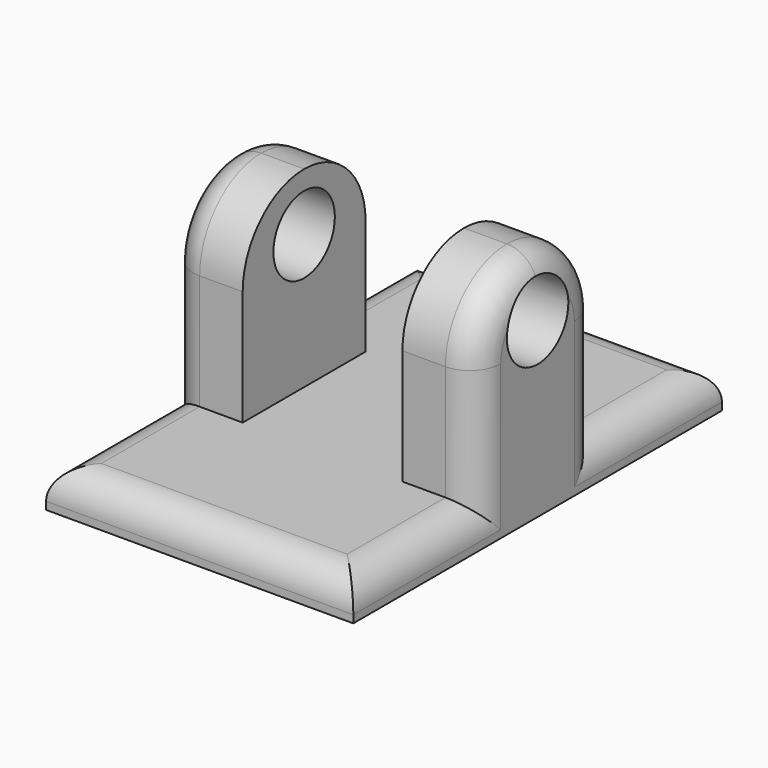
from build123d import *

# Parameters (mm, degrees)
F0_W         = 50.8
F0_H         = 76.2
F1_DEPTH     = 6.35
F2_W         = 12.192
F2_H         = 25.4
F3_DEPTH     = 31.75
F5_D         = 12.7
F5_DEPTH     = 254
F5_TIP       = 3.8154649308
F6_R         = 12.69999
F7_T1_DEPTH  = 19.05001
F7_T3_DEPTH  = 76.2
F7_T5_DEPTH  = 38.1
F7_T7_DEPTH  = 38.1
F7_T9_DEPTH  = 2e-05
F7_T12_ANGLE = 90
F7_T14_ANGLE = 90
F7_T16_ANGLE = 90
F7_T18_ANGLE = 90
F7_T23_DEPTH = 31.75001
F7_T28_DEPTH = 38.1
F7_T35_DEPTH = 38.1
F7_T39_DEPTH = 31.75001
F7_T47_DEPTH = 38.1
F7_T51_DEPTH = 31.75001
F7_T59_DEPTH = 31.75001
F7_T64_DEPTH = 38.1


# Not quite as in the source:
# - a fillet or chamfer that OpenCascade refuses, or shapes differently, is made with other operations: its cross-section is extruded or revolved along the edge and cut away or added
# - a fillet or chamfer is up to 0.001 mm smaller than in the source, because OpenCascade refuses the exact size


with BuildPart() as f1:
    # F0 (on Top) → F1 (new body)
    with BuildSketch(Plane.XY):
        Rectangle(F0_W, F0_H)
    extrude(amount=F1_DEPTH)

    # F2 (on face) → F3 (join)
    with BuildSketch(Plane.XY.offset(6.35)):
        with Locations((-19.304, 0)):
            Rectangle(F2_W, F2_H)
        with Locations((19.304, 0)):
            Rectangle(F2_W, F2_H)
    extrude(amount=F3_DEPTH)

    # F5
    with Locations(Plane(origin=(-25.4, 0, 0), x_dir=(0, -1, 0), z_dir=(-1, 0, 0))):
        with Locations((0, 28.575)):
            Hole(F5_D / 2, depth=F5_DEPTH)
            with Locations((0, 0, -(F5_DEPTH + F5_TIP / 2))):  # 118° drill point
                Cone(0, F5_D / 2, F5_TIP, mode=Mode.SUBTRACT)

    # F6 (radius 12.7 in the source; OpenCascade refuses exactly that, so slightly less here)
    f6_edges = [f1.edges().sort_by_distance(p)[0] for p in [
        (19.304, 12.7, 38.1),
        (19.304, -12.7, 38.1),
        (-19.304, 12.7, 38.1),
        (-19.304, -12.7, 38.1),
    ]]
    fillet(f6_edges, radius=F6_R)

    # F7: fillet of radius 5.08 on 14 edges, made by hand

    # F7_s2 → F7_t1 (cut)
    with BuildSketch(Plane.XY.offset(6.35)):
        with BuildLine():
            ThreePointArc((-25.4, 7.62), (-23.9121024484, 11.2121024484), (-20.32, 12.7))
            Line((-20.32, 12.7), (-25.4, 12.7))
            Line((-25.4, 12.7), (-25.4, 7.62))
        make_face()
        with BuildLine():
            ThreePointArc((25.4, -7.62), (23.9121024484, -11.2121024484), (20.32, -12.7))
            Line((20.32, -12.7), (25.4, -12.7))
            Line((25.4, -12.7), (25.4, -7.62))
        make_face()
        with BuildLine():
            ThreePointArc((-25.4, -7.62), (-23.9121024484, -11.2121024484), (-20.32, -12.7))
            Line((-20.32, -12.7), (-25.4, -12.7))
            Line((-25.4, -12.7), (-25.4, -7.62))
        make_face()
        with BuildLine():
            ThreePointArc((25.4, 7.62), (23.9121024484, 11.2121024484), (20.32, 12.7))
            Line((20.32, 12.7), (25.4, 12.7))
            Line((25.4, 12.7), (25.4, 7.62))
        make_face()
    extrude(amount=F7_T1_DEPTH, mode=Mode.SUBTRACT)

    # F7_s4 → F7_t3 (cut)
    with BuildSketch(Plane.YZ.offset(-38.1)):
        with BuildLine():
            ThreePointArc((-33.02, 6.35), (-36.6121024484, 4.8621024484), (-38.1, 1.27))
            Line((-38.1, 1.27), (-38.1, 6.35))
            Line((-38.1, 6.35), (-33.02, 6.35))
        make_face()
        with BuildLine():
            ThreePointArc((33.02, 6.35), (36.6121024484, 4.8621024484), (38.1, 1.27))
            Line((38.1, 1.27), (38.1, 6.35))
            Line((38.1, 6.35), (33.02, 6.35))
        make_face()
    extrude(amount=F7_T3_DEPTH, mode=Mode.SUBTRACT)

    # F7_s6 → F7_t5 (cut)
    with BuildSketch(Plane.XZ.offset(12.7)):
        with BuildLine():
            ThreePointArc((20.32, 6.35), (23.9121024484, 4.8621024484), (25.4, 1.27))
            Line((25.4, 1.27), (25.4, 6.35))
            Line((25.4, 6.35), (20.32, 6.35))
        make_face()
        with BuildLine():
            ThreePointArc((-25.4, 1.27), (-23.9121024484, 4.8621024484), (-20.32, 6.35))
            Line((-20.32, 6.35), (-25.4, 6.35))
            Line((-25.4, 6.35), (-25.4, 1.27))
        make_face()
    extrude(amount=F7_T5_DEPTH, mode=Mode.SUBTRACT)

    # F7_s8 → F7_t7 (cut)
    with BuildSketch(Plane.XZ.offset(-50.8)):
        with BuildLine():
            ThreePointArc((20.32, 6.35), (23.9121024484, 4.8621024484), (25.4, 1.27))
            Line((25.4, 1.27), (25.4, 6.35))
            Line((25.4, 6.35), (20.32, 6.35))
        make_face()
        with BuildLine():
            ThreePointArc((-25.4, 1.27), (-23.9121024484, 4.8621024484), (-20.32, 6.35))
            Line((-20.32, 6.35), (-25.4, 6.35))
            Line((-25.4, 6.35), (-25.4, 1.27))
        make_face()
    extrude(amount=F7_T7_DEPTH, mode=Mode.SUBTRACT)

    # F7_s10 → F7_t9 (cut)
    with BuildSketch(Plane.XZ.offset(-1e-05)):
        with BuildLine():
            ThreePointArc((25.4, 33.02), (23.9121024484, 36.6121024484), (20.32, 38.1))
            Line((20.32, 38.1), (25.4, 38.1))
            Line((25.4, 38.1), (25.4, 33.02))
        make_face()
        with BuildLine():
            ThreePointArc((-25.4, 33.02), (-23.9121024484, 36.6121024484), (-20.32, 38.1))
            Line((-20.32, 38.1), (-25.4, 38.1))
            Line((-25.4, 38.1), (-25.4, 33.02))
        make_face()
    extrude(amount=F7_T9_DEPTH, mode=Mode.SUBTRACT)

    # F7_s11 → F7_t12 (revolve, cut)
    with BuildSketch(Plane.XY.offset(25.40001)):
        with BuildLine():
            ThreePointArc((-25.4, 7.62), (-23.9121024484, 11.2121024484), (-20.32, 12.7))
            Line((-20.32, 12.7), (-25.4, 12.7))
            Line((-25.4, 12.7), (-25.4, 7.62))
        make_face()
    revolve(axis=Axis((-25.4, 1e-05, 25.40001), (1, 0, 0)), revolution_arc=F7_T12_ANGLE, mode=Mode.SUBTRACT)

    # F7_s13 → F7_t14 (revolve, cut)
    with BuildSketch(Plane.XZ.offset(1e-05)):
        with BuildLine():
            ThreePointArc((-25.4, 33.02), (-23.9121024484, 36.6121024484), (-20.32, 38.1))
            Line((-20.32, 38.1), (-25.4, 38.1))
            Line((-25.4, 38.1), (-25.4, 33.02))
        make_face()
    revolve(axis=Axis((-25.4, -1e-05, 25.40001), (1, 0, 0)), revolution_arc=F7_T14_ANGLE, mode=Mode.SUBTRACT)

    # F7_s15 → F7_t16 (revolve, cut)
    with BuildSketch(Plane.XY.offset(25.40001)):
        with BuildLine():
            ThreePointArc((25.4, -7.62), (23.9121024484, -11.2121024484), (20.32, -12.7))
            Line((20.32, -12.7), (25.4, -12.7))
            Line((25.4, -12.7), (25.4, -7.62))
        make_face()
    revolve(axis=Axis((25.4, -1e-05, 25.40001), (-1, 0, 0)), revolution_arc=F7_T16_ANGLE, mode=Mode.SUBTRACT)

    # F7_s17 → F7_t18 (revolve, cut)
    with BuildSketch(Plane.XZ.offset(-1e-05)):
        with BuildLine():
            ThreePointArc((25.4, 33.02), (23.9121024484, 36.6121024484), (20.32, 38.1))
            Line((20.32, 38.1), (25.4, 38.1))
            Line((25.4, 38.1), (25.4, 33.02))
        make_face()
    revolve(axis=Axis((25.4, 1e-05, 25.40001), (-1, 0, 0)), revolution_arc=F7_T18_ANGLE, mode=Mode.SUBTRACT)


with BuildPart() as f7_tool21:
    # F7_s22 → F7_t23 (new body)
    with BuildSketch(Plane.XY.offset(-6.35)):
        with BuildLine():
            ThreePointArc((-25.4, 7.62), (-23.9121024484, 11.2121024484), (-20.32, 12.7))
            Line((-20.32, 12.7), (-25.4, 12.7))
            Line((-25.4, 12.7), (-25.4, 7.62))
        make_face()
    extrude(amount=F7_T23_DEPTH)

    split(bisect_by=Plane.XY.offset(6.35), keep=Keep.BOTTOM)

    split(bisect_by=Plane.XY, keep=Keep.TOP)


with BuildPart() as f7_tool26:
    # F7_s27 → F7_t28 (new body)
    with BuildSketch(Plane.XZ.offset(-38.1)):
        with BuildLine():
            ThreePointArc((-25.4, 1.27), (-23.9121024484, 4.8621024484), (-20.32, 6.35))
            Line((-20.32, 6.35), (-25.4, 6.35))
            Line((-25.4, 6.35), (-25.4, 1.27))
        make_face()
    extrude(amount=F7_T28_DEPTH)

    split(bisect_by=Plane.XZ.offset(-12.7), keep=Keep.TOP)


with BuildPart() as f7_tool21_1:
    add(f7_tool21.part)

    # F7_t30: intersect F7_tool26
    add(f7_tool26.part, mode=Mode.INTERSECT)


with BuildPart() as f1_1:
    add(f1.part)

    # F7_t19: cut F7_tool21
    add(f7_tool21_1.part, mode=Mode.SUBTRACT)


with BuildPart() as f7_tool33:
    # F7_s34 → F7_t35 (new body)
    with BuildSketch(Plane.XZ.offset(38.1)):
        with BuildLine():
            ThreePointArc((20.32, 6.35), (23.9121024484, 4.8621024484), (25.4, 1.27))
            Line((25.4, 1.27), (25.4, 6.35))
            Line((25.4, 6.35), (20.32, 6.35))
        make_face()
    extrude(amount=-F7_T35_DEPTH)

    split(bisect_by=Plane.XZ.offset(12.7), keep=Keep.BOTTOM)


with BuildPart() as f7_tool37:
    # F7_s38 → F7_t39 (new body)
    with BuildSketch(Plane.XY.offset(-6.35)):
        with BuildLine():
            ThreePointArc((25.4, -7.62), (23.9121024484, -11.2121024484), (20.32, -12.7))
            Line((20.32, -12.7), (25.4, -12.7))
            Line((25.4, -12.7), (25.4, -7.62))
        make_face()
    extrude(amount=F7_T39_DEPTH)

    split(bisect_by=Plane.XY.offset(6.35), keep=Keep.BOTTOM)

    split(bisect_by=Plane.XY, keep=Keep.TOP)


with BuildPart() as f7_tool33_1:
    add(f7_tool33.part)

    # F7_t42: intersect F7_tool37
    add(f7_tool37.part, mode=Mode.INTERSECT)


with BuildPart() as f1_2:
    add(f1_1.part)

    # F7_t31: cut F7_tool33
    add(f7_tool33_1.part, mode=Mode.SUBTRACT)


with BuildPart() as f7_tool45:
    # F7_s46 → F7_t47 (new body)
    with BuildSketch(Plane.XZ):
        with BuildLine():
            ThreePointArc((20.32, 6.35), (23.9121024484, 4.8621024484), (25.4, 1.27))
            Line((25.4, 1.27), (25.4, 6.35))
            Line((25.4, 6.35), (20.32, 6.35))
        make_face()
    extrude(amount=-F7_T47_DEPTH)

    split(bisect_by=Plane.XZ.offset(-12.7), keep=Keep.TOP)


with BuildPart() as f7_tool49:
    # F7_s50 → F7_t51 (new body)
    with BuildSketch(Plane.XY.offset(-6.35)):
        with BuildLine():
            ThreePointArc((25.4, 7.62), (23.9121024484, 11.2121024484), (20.32, 12.7))
            Line((20.32, 12.7), (25.4, 12.7))
            Line((25.4, 12.7), (25.4, 7.62))
        make_face()
    extrude(amount=F7_T51_DEPTH)

    split(bisect_by=Plane.XY.offset(6.35), keep=Keep.BOTTOM)

    split(bisect_by=Plane.XY, keep=Keep.TOP)


with BuildPart() as f7_tool45_1:
    add(f7_tool45.part)

    # F7_t54: intersect F7_tool49
    add(f7_tool49.part, mode=Mode.INTERSECT)


with BuildPart() as f1_3:
    add(f1_2.part)

    # F7_t43: cut F7_tool45
    add(f7_tool45_1.part, mode=Mode.SUBTRACT)


with BuildPart() as f7_tool57:
    # F7_s58 → F7_t59 (new body)
    with BuildSketch(Plane.XY.offset(-6.35)):
        with BuildLine():
            ThreePointArc((-25.4, -7.62), (-23.9121024484, -11.2121024484), (-20.32, -12.7))
            Line((-20.32, -12.7), (-25.4, -12.7))
            Line((-25.4, -12.7), (-25.4, -7.62))
        make_face()
    extrude(amount=F7_T59_DEPTH)

    split(bisect_by=Plane.XY.offset(6.35), keep=Keep.BOTTOM)

    split(bisect_by=Plane.XY, keep=Keep.TOP)


with BuildPart() as f7_tool62:
    # F7_s63 → F7_t64 (new body)
    with BuildSketch(Plane.XZ):
        with BuildLine():
            ThreePointArc((-25.4, 1.27), (-23.9121024484, 4.8621024484), (-20.32, 6.35))
            Line((-20.32, 6.35), (-25.4, 6.35))
            Line((-25.4, 6.35), (-25.4, 1.27))
        make_face()
    extrude(amount=F7_T64_DEPTH)

    split(bisect_by=Plane.XZ.offset(12.7), keep=Keep.BOTTOM)


with BuildPart() as f7_tool57_1:
    add(f7_tool57.part)

    # F7_t66: intersect F7_tool62
    add(f7_tool62.part, mode=Mode.INTERSECT)


with BuildPart() as f1_4:
    add(f1_3.part)

    # F7_t55: cut F7_tool57
    add(f7_tool57_1.part, mode=Mode.SUBTRACT)


solid = f1_4.part
